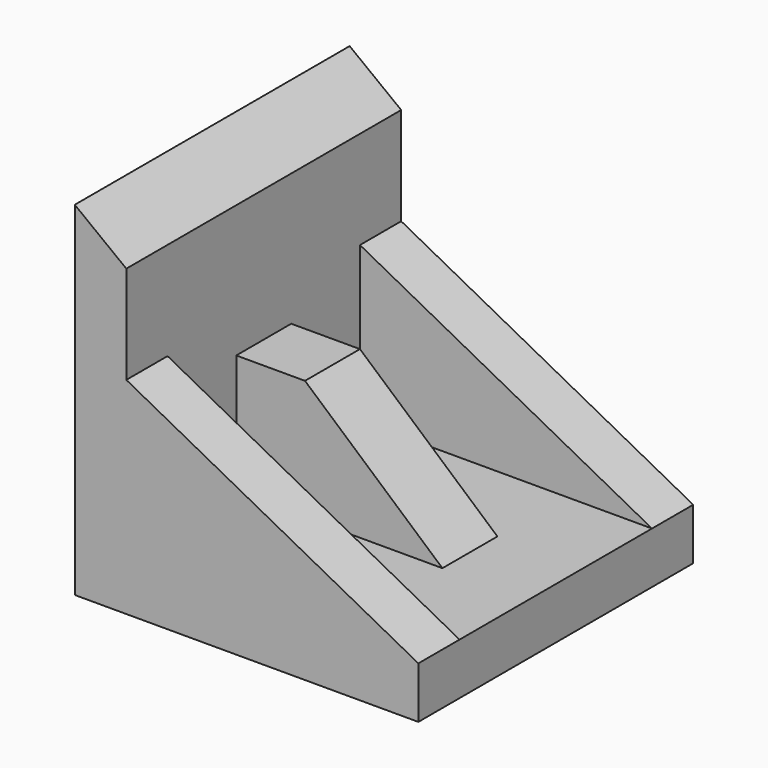
from build123d import *

# Parameters (mm, degrees)
F1_DEPTH = 127
F3_DEPTH = 38.1
F4_DEPTH = 25.4


# Not quite as in the source:
# - a pattern or mirror of a feature is missing from the dataset's text; its kind, count and spacing are read off the source's solid


with BuildPart() as f1:
    # F0 (on Front) → F1 (new body, symmetric)
    with BuildSketch(Plane.XZ):
        Polygon((0, 88.9), (0, 186.69), (-38.1, 215.9), (-38.1, -38.1), (215.9, -38.1), (215.9, 0), (152.4, 0), (0, 0), align=None)
    extrude(amount=F1_DEPTH, both=True)

    # F2 (on face) → F3 (join)
    with BuildSketch(Plane.XZ.offset(127)):
        Polygon((215.9, 0), (0, 114.3), (0, 0), align=None)
    f3 = extrude(amount=-F3_DEPTH)

    # F3_copies: F3 across plane
    add(f3.mirror(Plane.ZX))

    # F0 (on Front) → F4 (join, symmetric)
    with BuildSketch(Plane.XZ):
        Polygon((0, 88.9), (0, 186.69), (-38.1, 215.9), (-38.1, -38.1), (215.9, -38.1), (215.9, 0), (152.4, 0), (0, 0), align=None)
        Polygon((50.8, 88.9), (0, 88.9), (0, 0), (152.4, 0), align=None)
    extrude(amount=F4_DEPTH, both=True)


solid = f1.part
